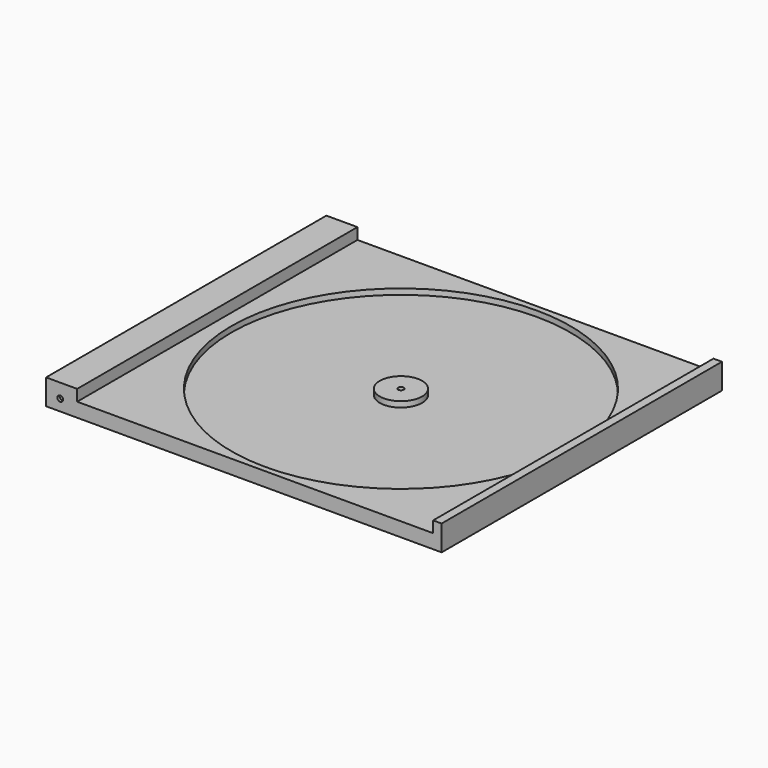
from build123d import *

# Parameters (mm, degrees)
F0_W     = 126
F0_H     = 124
F0_W_2   = 11
F0_W_3   = 3
F1_DEPTH = 5
F2_DEPTH = 9
F3_R     = 60
F3_R_2   = 7.5
F4_DEPTH = 2
F5_R     = 1
F6_DEPTH = 2
F7_R     = 1
F8_DEPTH = 1


# Not quite as in the source:
# - a feature names something its author has since deleted; it is built from what else it names


with BuildPart() as f1:
    # F0 (on Top) → F1 (new body)
    with BuildSketch(Plane.XY):
        with Locations((4, 0)):
            Rectangle(F0_W, F0_H)
        with Locations((-64.5, 0)):
            Rectangle(F0_W_2, F0_H)
        with Locations((68.5, 0)):
            Rectangle(F0_W_3, F0_H)
    extrude(amount=F1_DEPTH)

    # F0 (on Top) → F2 (join)
    with BuildSketch(Plane.XY):
        with Locations((-64.5, 0)):
            Rectangle(F0_W_2, F0_H)
        with Locations((68.5, 0)):
            Rectangle(F0_W_3, F0_H)
    extrude(amount=F2_DEPTH)

    # F3 (on face) → F4 (cut)
    with BuildSketch(Plane.XY.offset(5)):
        with Locations((6.0000000522, 0)):
            Circle(F3_R)
        with Locations((6.0000000522, 0)):
            Circle(F3_R_2, mode=Mode.SUBTRACT)
    extrude(amount=-F4_DEPTH, mode=Mode.SUBTRACT)

    # F5 (on face) → F6 (cut)
    with BuildSketch(Plane.XY.offset(5)):
        with Locations((6.0000000522, 0)):
            Circle(F5_R)
    extrude(amount=-F6_DEPTH, mode=Mode.SUBTRACT)

    # F7 (on face) → F8 (cut)
    with BuildSketch(Plane.XZ.offset(62)):
        with Locations((-64.9999976158, 4)):
            Circle(F7_R)
    extrude(amount=-F8_DEPTH, mode=Mode.SUBTRACT)


solid = f1.part
